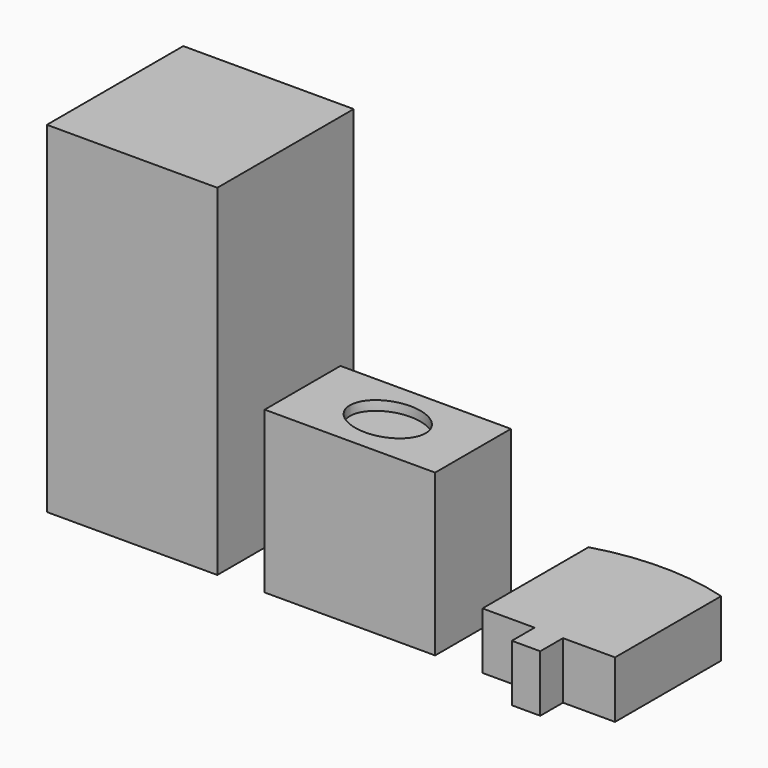
from build123d import *

# Parameters (mm, degrees)
F0_W     = 914.4
F0_H     = 914.4
F1_DEPTH = 1828.8
F2_W     = 914.4
F2_H     = 508
F3_DEPTH = 863.6
F5_DEPTH = 50.8
F7_DEPTH = 304.8


# Not quite as in the source:
# - a feature of the source that left no trace in its solid (it failed there, or was rolled back) is left out


with BuildPart() as f1:
    # F0 (on Top) → F1 (new body)
    with BuildSketch(Plane.XY):
        with Locations((457.2, 457.2)):
            Rectangle(F0_W, F0_H)
    extrude(amount=F1_DEPTH)


with BuildPart() as f3:
    # F2 (on Top) → F3 (new body)
    with BuildSketch(Plane.XY):
        with Locations((1625.6, 254)):
            Rectangle(F2_W, F2_H)
    extrude(amount=F3_DEPTH)

    # F4 (on face) → F5 (cut)
    with BuildSketch(Plane.XY.offset(863.6)):
        with BuildLine():
            add(Edge.make_bspline(
                [(1828.8, 254), (1828.8, 406.4), (1625.6, 406.4)],
                knots=[0, 0, 0, 1.5707963268, 1.5707963268, 1.5707963268], degree=2, weights=[1, 0.7071067812, 1]))
            Line((1625.6, 406.4), (1625.6, 254))
            Line((1625.6, 254), (1828.8, 254))
        make_face()
        with BuildLine():
            Line((1625.6, 254), (1625.6, 406.4))
            add(Edge.make_bspline(
                [(1625.6, 406.4), (1422.4, 406.4), (1422.4, 254)],
                knots=[1.5707963268, 1.5707963268, 1.5707963268, 3.1415926536, 3.1415926536, 3.1415926536], degree=2, weights=[1, 0.7071067812, 1]))
            Line((1422.4, 254), (1625.6, 254))
        make_face()
        with BuildLine():
            Line((1828.8, 254), (1625.6, 254))
            Line((1625.6, 254), (1625.6, 101.6))
            add(Edge.make_bspline(
                [(1625.6, 101.6), (1828.8, 101.6), (1828.8, 254)],
                knots=[4.7123889804, 4.7123889804, 4.7123889804, 6.2831853072, 6.2831853072, 6.2831853072], degree=2, weights=[1, 0.7071067812, 1]))
        make_face()
        with BuildLine():
            Line((1625.6, 101.6), (1625.6, 254))
            Line((1625.6, 254), (1422.4, 254))
            add(Edge.make_bspline(
                [(1422.4, 254), (1422.4, 101.6), (1625.6, 101.6)],
                knots=[3.1415926536, 3.1415926536, 3.1415926536, 4.7123889804, 4.7123889804, 4.7123889804], degree=2, weights=[1, 0.7071067812, 1]))
        make_face()
    extrude(amount=-F5_DEPTH, mode=Mode.SUBTRACT)


with BuildPart() as f7:
    # F6 (on Top) → F7 (new body)
    with BuildSketch(Plane.XY):
        with BuildLine():
            Line((2336.8, 711.2), (2336.8, 0))
            Line((2336.8, 0), (2616.2, 0))
            Line((2616.2, 0), (2616.2, -152.4))
            Line((2616.2, -152.4), (2692.4, -152.4))
            Line((2692.4, -152.4), (2692.4, 762))
            ThreePointArc((2692.4, 762), (2512.7948775786, 749.2358569497), (2336.8, 711.2))
        make_face()
        with BuildLine():
            ThreePointArc((3048, 711.2), (2872.0051224214, 749.2358569497), (2692.4, 762))
            Line((2692.4, 762), (2692.4, -152.4))
            Line((2692.4, -152.4), (2768.6, -152.4))
            Line((2768.6, -152.4), (2768.6, 0))
            Line((2768.6, 0), (3048, 0))
            Line((3048, 0), (3048, 711.2))
        make_face()
    extrude(amount=F7_DEPTH)


solid = Compound([f1.part, f3.part, f7.part])
